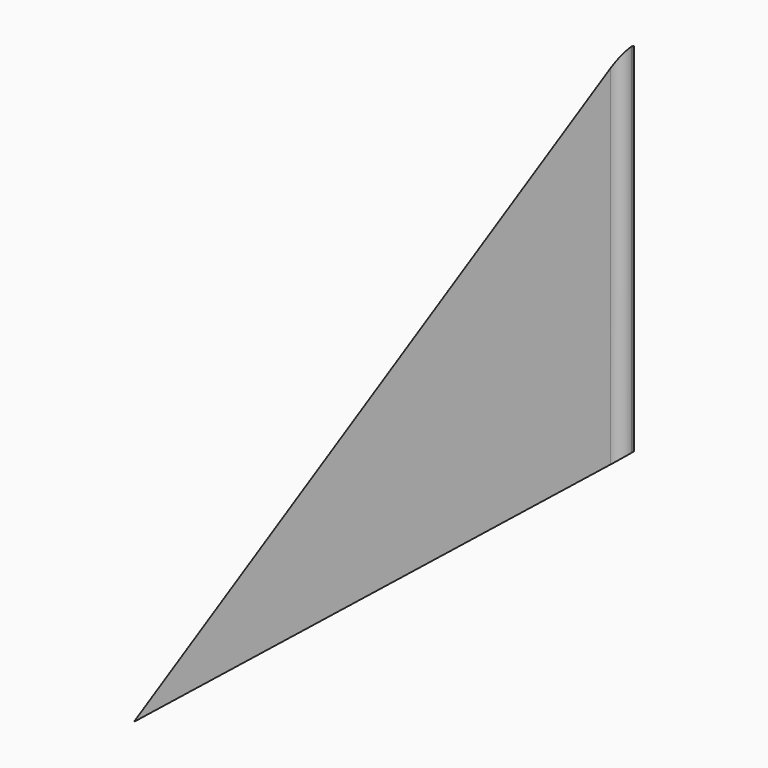
from build123d import *

# Parameters (mm, degrees)
F1_DEPTH    = 2.5
F2_T1_DEPTH = 46.75


# Not quite as in the source:
# - a fillet or chamfer that OpenCascade refuses, or shapes differently, is made with other operations: its cross-section is extruded or revolved along the edge and cut away or added


with BuildPart() as f1:
    # F0 (on Front) → F1 (new body)
    with BuildSketch(Plane.XZ):
        Polygon((-54.643732486, -43.75), (0, 0), (0, 40), align=None)
    extrude(amount=F1_DEPTH)

    # F2: fillet of radius 1.35 on 2 edges, made by hand

    # F2_s2 → F2_t1 (cut)
    with BuildSketch(Plane.XY.offset(-3.375)):
        with BuildLine():
            ThreePointArc((0, -1.15), (-0.3954058454, -2.1045941546), (-1.35, -2.5))
            Line((-1.35, -2.5), (0, -2.5))
            Line((0, -2.5), (0, -1.15))
        make_face()
        with BuildLine():
            ThreePointArc((0, -1.35), (-0.3954058454, -0.3954058454), (-1.35, 0))
            Line((-1.35, 0), (0, 0))
            Line((0, 0), (0, -1.35))
        make_face()
    extrude(amount=F2_T1_DEPTH, mode=Mode.SUBTRACT)


solid = f1.part
